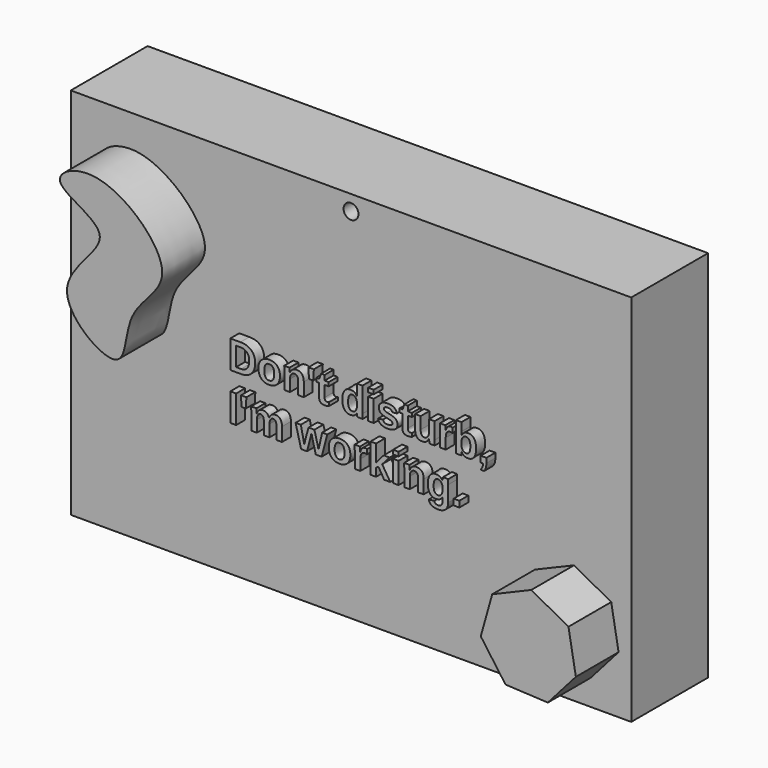
from build123d import *

# Parameters (mm, degrees)
F0_W         = 150
F0_H         = 100
F1_DEPTH     = 0.7
F3_DEPTH     = 25
F4_DEPTH     = 40
F5_TEXT_SIZE = 10.8340789824
F6_DEPTH     = 3
F7_R         = 2
F8_DEPTH     = 25.7


# Not quite as in the source:
# - Text() gives the source's letters only with a copy of the font that has no kerning and outlines rounded to 1/6400 em; it was checked with that copy


with BuildPart() as f1:
    # F0 (on Front) → F1 (new body)
    with BuildSketch(Plane.XZ):
        Rectangle(F0_W, F0_H)
    extrude(amount=F1_DEPTH)

    # F3 (add): a face of the model
    f3_faces = [f1.faces().sort_by_distance(p)[0] for p in [
        (0, -0.7, 0),
    ]]
    extrude(f3_faces, amount=F3_DEPTH)

    # F2 (on Front) → F4 (join)
    with BuildSketch(Plane.XZ):
        with BuildLine():
            add(Edge.make_bspline(
                [(-66.3539245725, 37.038680166), (-65.3258824298, 34.2478528529), (-46.6130320141, 28.8186600601), (-73.9876621266, 12.7371800573), (-47.5922253117, -6.6099133978), (-50.0444909227, 13.8875224689), (-31.5817151118, 23.7137547662), (-55.1211003875, 46.0373868231), (-67.2335992772, 39.4267342066), (-66.3539245725, 37.038680166)],
                knots=[0, 0, 0, 0, 0.1337134012, 0.2877315462, 0.4390632136, 0.5658030643, 0.707304533, 0.8855841684, 1, 1, 1, 1], degree=3))
        make_face()
        Polygon((59.6806322025, -18.0807772203), (49.2339001887, -22.489189622), (46.1671049188, -33.4053737741), (52.7896057821, -42.6092203606), (64.1145245543, -43.1700451774), (71.6139664136, -34.6655356989), (69.6406986792, -23.4997610227), align=None)
    extrude(amount=F4_DEPTH)

    # F5 (on face) → F6 (join)
    with BuildSketch(Plane.XZ.offset(25.7)):
        with Locations((-30.6265463106, 0)):
            Text("Don't disturb,", F5_TEXT_SIZE, font='Arimo', font_style=FontStyle.BOLD, text_align=(TextAlign.LEFT, TextAlign.BOTTOM))
        with Locations((-30.6265463106, -12.4591908297)):
            Text("I'm working.", F5_TEXT_SIZE, font='Arimo', font_style=FontStyle.BOLD, text_align=(TextAlign.LEFT, TextAlign.BOTTOM))
    extrude(amount=F6_DEPTH)

    # F7 (on face) → F8 (cut, through all)
    with BuildSketch(Plane.XZ.offset(25.7)):
        with Locations((0, 45.8764458142)):
            Circle(F7_R)
    extrude(amount=-F8_DEPTH, mode=Mode.SUBTRACT)


solid = f1.part
